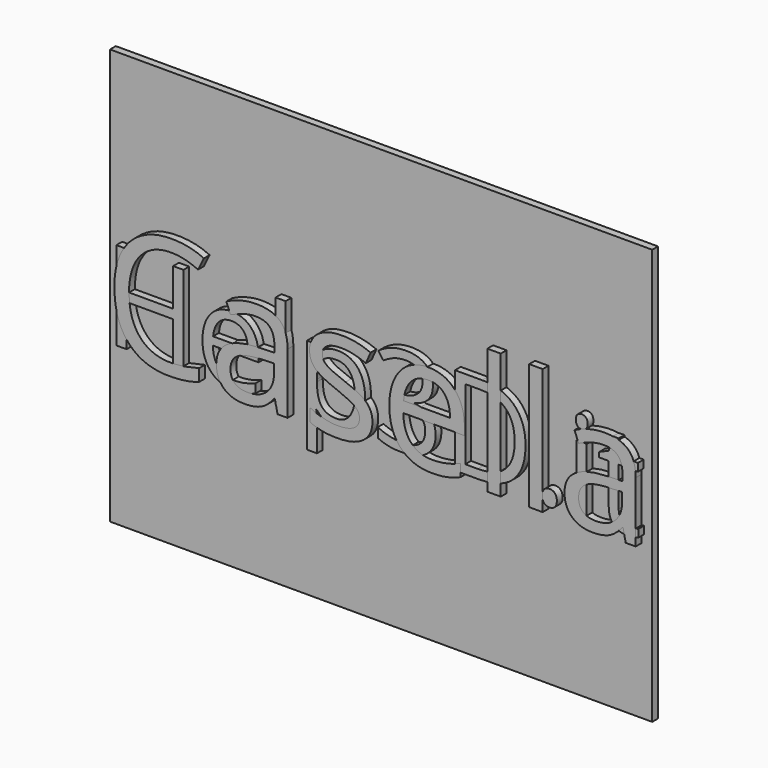
from build123d import *

# Parameters (mm, degrees)
F0_W         = 150
F0_H         = 115
F1_DEPTH     = 2
F2_TEXT_SIZE = 34.2355836097
F3_DEPTH     = 2
F4_DEPTH     = 2
F5_TEXT_SIZE = 45.8562216384
F6_DEPTH     = 2


# Not quite as in the source:
# - Text() gives the source's letters only with a copy of the font that has no kerning and outlines rounded to 1/6400 em; it was checked with that copy


with BuildPart() as f1:
    # F0 (on Front) → F1 (new body)
    with BuildSketch(Plane.XZ):
        Rectangle(F0_W, F0_H)
    extrude(amount=F1_DEPTH)

    # F2 (on face) → F3 (join)
    with BuildSketch(Plane.XZ.offset(2)):
        with Locations((-75, -12.6897491472)):
            Text('Help3D.it', F2_TEXT_SIZE, font='Open Sans', text_align=(TextAlign.LEFT, TextAlign.BOTTOM))
    extrude(amount=F3_DEPTH)


with BuildPart() as f4:
    # F0 (on Front) → F4 (new body)
    with BuildSketch(Plane.XZ):
        Rectangle(F0_W, F0_H)
    extrude(amount=F4_DEPTH)

    # F5 (on face) → F6 (join)
    with BuildSketch(Plane.XZ.offset(2)):
        with Locations((-75, -14.9349922146)):
            Text('Casella', F5_TEXT_SIZE, font='Open Sans', text_align=(TextAlign.LEFT, TextAlign.BOTTOM))
    extrude(amount=F6_DEPTH)


solid = Compound([f1.part, f4.part])
